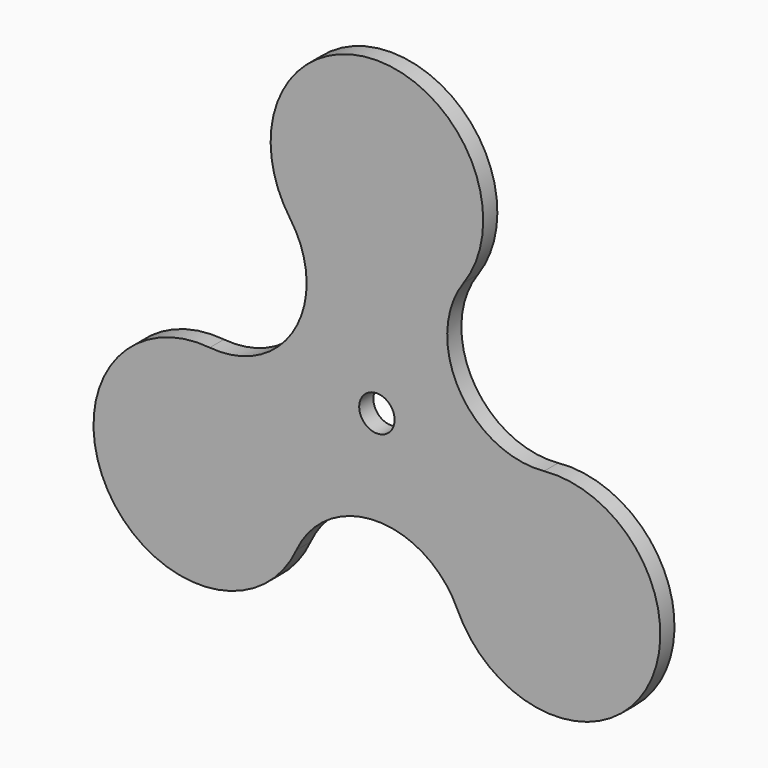
from build123d import *

# Parameters (mm, degrees)
F0_R     = 2.54
F1_DEPTH = 2.54
F2_R     = 10.16
F3_DEPTH = 1.27


# Not quite as in the source:
# - a feature names something its author has since deleted; it is built from what else it names


with BuildPart() as f1:
    # F0 (on Front) → F1 (new body)
    with BuildSketch(Plane.XZ):
        with BuildLine():
            ThreePointArc((23.9710795428, 0.5081666473), (11.7817898671, 6.8022195513), (12.4256249974, 20.5054805165))
            ThreePointArc((12.4256249974, 20.5054805165), (0, 44.5693936748), (-12.4256249974, 20.5054805165))
            ThreePointArc((-12.4256249974, 20.5054805165), (-11.7817898671, 6.8022195513), (-23.9710795428, 0.5081666473))
            ThreePointArc((-23.9710795428, 0.5081666473), (-38.5982271537, -22.2846968374), (-11.5454545455, -21.0136471639))
            ThreePointArc((-11.5454545455, -21.0136471639), (0, -13.6044391026), (11.5454545455, -21.0136471639))
            ThreePointArc((11.5454545455, -21.0136471639), (38.5982271537, -22.2846968374), (23.9710795428, 0.5081666473))
        make_face()
        Circle(F0_R, mode=Mode.SUBTRACT)
    extrude(amount=F1_DEPTH)

    # F2 (on face) → F3 (cut)
    with BuildSketch(Plane(origin=(0, 0, 0), x_dir=(-1, 0, 0), z_dir=(0, 1, 0))):
        with Locations((25.4, -14.6646968374)):
            Circle(F2_R)
        with Locations((0, 29.3293936748)):
            Circle(F2_R)
        with Locations((-25.4, -14.6646968374)):
            Circle(F2_R)
    extrude(amount=-F3_DEPTH, mode=Mode.SUBTRACT)


solid = f1.part
